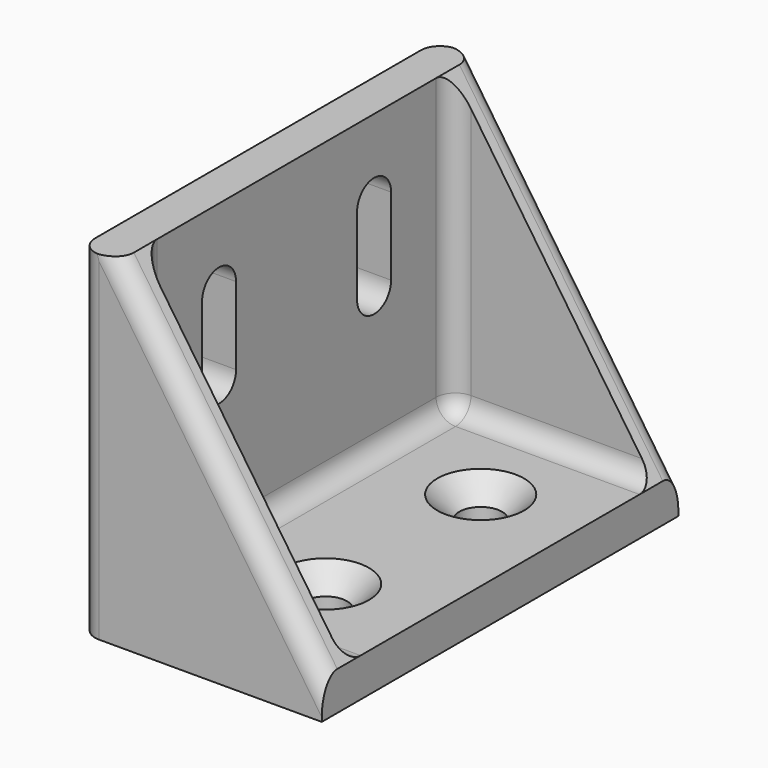
from build123d import *

# Parameters (mm, degrees)
F1_DEPTH       = 40
F3_DEPTH       = 4
F5_D           = 4.4
F5_CSINK_D     = 8.96
F5_CSINK_ANGLE = 90
F7_DEPTH       = 3
F10_R          = 2
F11_T1_DEPTH   = 45


# Not quite as in the source:
# - a fillet or chamfer that OpenCascade refuses, or shapes differently, is made with other operations: its cross-section is extruded or revolved along the edge and cut away or added


with BuildPart() as f1:
    # F0 (on Front) → F1 (new body)
    with BuildSketch(Plane.XZ):
        Polygon((-12.4999986735, 17.5), (-12.4999986735, -17.5), (12.4999986735, -17.5), (12.4999986735, -13.5), (-8.4999986735, -13.5), (-8.4999986735, 17.5), align=None)
    extrude(amount=F1_DEPTH)

    # F2 (on face) → F3 (cut, through all)
    with BuildSketch(Plane.YZ.offset(-8.4999986735)):
        with BuildLine():
            ThreePointArc((-27.8069023984, 9.5), (-30, 11.6930976016), (-32.1930976016, 9.5))
            Line((-32.1930976016, 9.5), (-32.1930976016, 1.5))
            ThreePointArc((-32.1930976016, 1.5), (-30, -0.6930976016), (-27.8069023984, 1.5))
            Line((-27.8069023984, 1.5), (-27.8069023984, 9.5))
        make_face()
        with BuildLine():
            Line((-7.8069023984, 1.5), (-7.8069023984, 9.5))
            ThreePointArc((-7.8069023984, 9.5), (-10, 11.6930976016), (-12.1930976016, 9.5))
            Line((-12.1930976016, 9.5), (-12.1930976016, 1.5))
            ThreePointArc((-12.1930976016, 1.5), (-10, -0.6930976016), (-7.8069023984, 1.5))
        make_face()
    extrude(amount=-F3_DEPTH, mode=Mode.SUBTRACT)

    # F5 (through all)
    with Locations(Plane.XY.offset(-13.5)):
        with Locations((2.4999986735, -30), (2.4999986735, -10)):
            CounterSinkHole(F5_D / 2, F5_CSINK_D / 2, counter_sink_angle=F5_CSINK_ANGLE)

    # F6 (on face) → F7 (join)
    with BuildSketch(Plane.XZ.offset(40)):
        Polygon((12.4999986735, -13.5), (-8.4999986735, 17.5), (-12.4999986735, 17.5), (-12.4999986735, -17.5), (12.4999986735, -17.5), align=None)
    extrude(amount=F7_DEPTH)

    # F9: F1 across plane


with BuildPart() as f1_1:
    add(f1.part)
    add(f1.part.mirror(Plane(origin=(-5.812499541, -20, -5.812499541), x_dir=(1, 0, 0), z_dir=(0, 1, 0))))

    # F10
    f10_edges = [f1_1.edges().sort_by_distance(p)[0] for p in [
        (-8.499999, -40, 2),
        (2, -40, -13.5),
        (-8.499999, -20, -13.5),
        (2, 0, -13.5),
        (-8.499999, 0, 2),
        (2, 3, 2),
        (2, -43, 2),
    ]]
    fillet(f10_edges, radius=F10_R)

    # F11: fillet of radius 2 on 2 edges, made by hand

    # F11_s2 → F11_t1 (cut)
    with BuildSketch(Plane.XY.offset(-22.5)):
        with BuildLine():
            ThreePointArc((-10.4999986735, 3), (-11.9142122359, 2.4142135624), (-12.4999986735, 1))
            Line((-12.4999986735, 1), (-12.4999986735, 3))
            Line((-12.4999986735, 3), (-10.4999986735, 3))
        make_face()
        with BuildLine():
            ThreePointArc((-12.4999986735, -41), (-11.9142122359, -42.4142135624), (-10.4999986735, -43))
            Line((-10.4999986735, -43), (-12.4999986735, -43))
            Line((-12.4999986735, -43), (-12.4999986735, -41))
        make_face()
    extrude(amount=F11_T1_DEPTH, mode=Mode.SUBTRACT)


solid = f1_1.part
